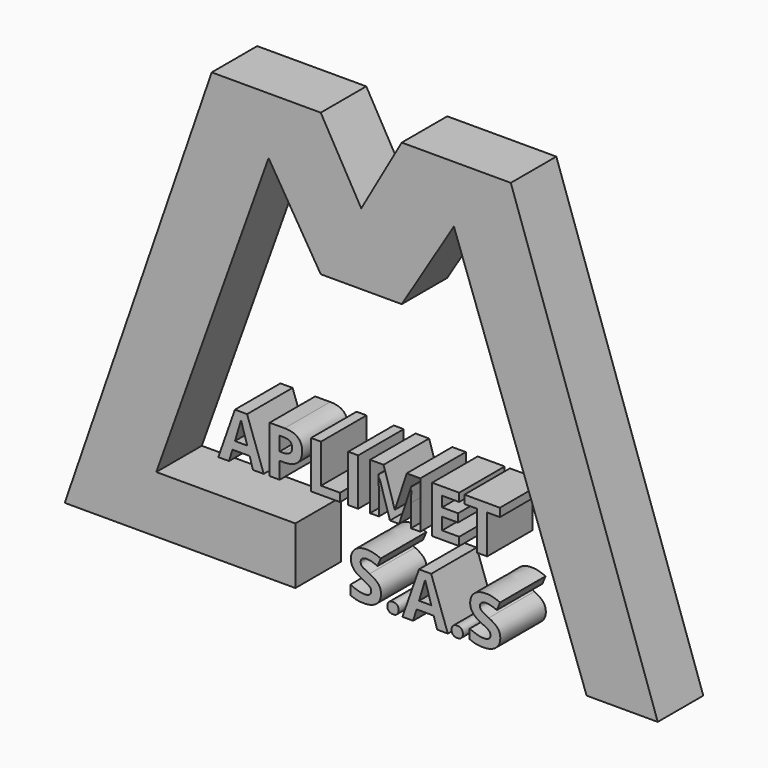
from build123d import *

# Parameters (mm, degrees)
F1_DEPTH     = 12
F2_TEXT_SIZE = 13.8888888889
F3_DEPTH     = 12
F5_SCALE     = 3


# Not quite as in the source:
# - Text() gives the source's letters only with a copy of the font that has no kerning and outlines rounded to 1/6400 em; it was checked with that copy


with BuildPart() as f1:
    # F0 (on Front) → F1 (new body)
    with BuildSketch(Plane.XZ):
        Polygon((-31.539775, 56.6728526354), (-62.5292601961, -33.3271473646), (-13.8875097036, -33.3271473646), (-13.8875097036, -21.3271473646), (-43.2231855505, -21.3271473646), (-19.539775, 44.6728526354), (-8.539775, 26.6728526354), (0, 26.6728526354), (8.5397779776, 26.6728526354), (19.5397779776, 44.6728526354), (47.5292631736, -33.3271473646), (62.5292631736, -33.3271473646), (31.5397779776, 56.6728526354), (8.5397779776, 56.6728526354), (0, 41.6728526354), (-8.539775, 56.6728526354), align=None)
    extrude(amount=-F1_DEPTH)


with BuildPart() as f3:
    # F2 (on face) → F3 (new body)
    with BuildSketch(Plane.XZ):
        with Locations((-30.1443142361, -14.3047785209)):
            Text('APLIMET', F2_TEXT_SIZE, font='Open Sans', font_style=FontStyle.BOLD, text_align=(TextAlign.LEFT, TextAlign.BOTTOM))
        with Locations((-2.9319880108, -31.3271473646)):
            Text('S.A.S', F2_TEXT_SIZE, font='Open Sans', font_style=FontStyle.BOLD, text_align=(TextAlign.LEFT, TextAlign.BOTTOM))
    extrude(amount=-F3_DEPTH)


with BuildPart() as f1_1:
    # F5: moved
    add(f1.part.scale(F5_SCALE))


with BuildPart() as f3_1:
    # F5: moved
    add(f3.part.scale(F5_SCALE))


solid = Compound([f1_1.part, f3_1.part])
